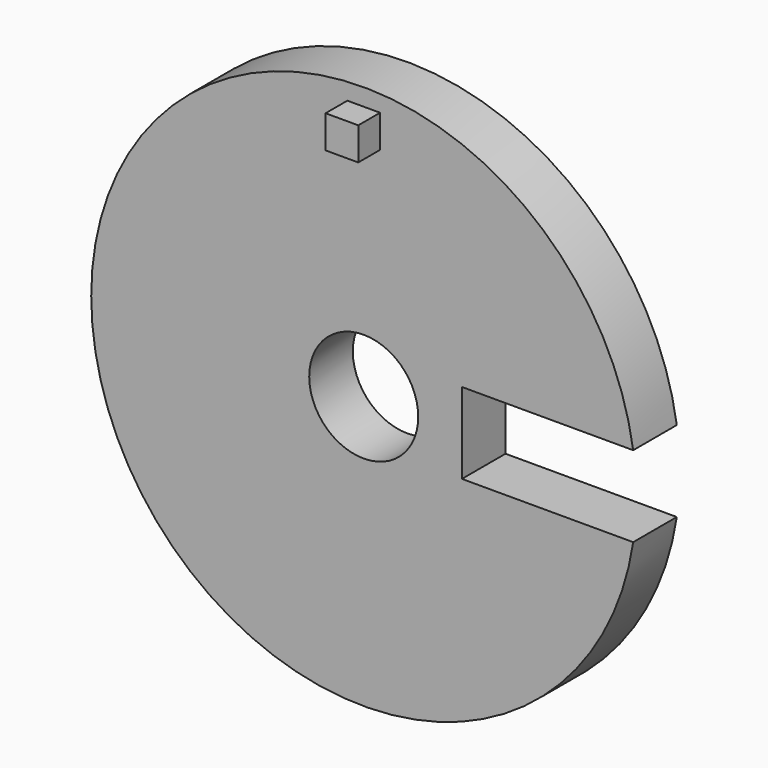
from build123d import *

# Parameters (mm, degrees)
F0_W     = 30
F0_H     = 60
F1_DEPTH = 100
F2_DEPTH = 102
F4_DEPTH = 100
F5_DEPTH = 150


# Not quite as in the source:
# - a feature of the source that left no trace in its solid (it failed there, or was rolled back) is left out
# - a feature names something its author has since deleted; it is built from what else it names


with BuildPart() as f1:
    # F0 (on Front) → F1 (new body)
    with BuildSketch(Plane.XZ):
        with BuildLine():
            Line((180.2002936602, 74.2409452796), (494.457563441, 74.2409452796))
            ThreePointArc((494.457563441, 74.2409452796), (326.2510746037, 378.8934366282), (0, 500))
            Line((0, 500), (0, 468.3614957333))
            Line((0, 468.3614957333), (30, 468.3614957333))
            Line((30, 468.3614957333), (30, 408.3614957333))
            Line((30, 408.3614957333), (0, 408.3614957333))
            Line((0, 408.3614957333), (0, 100))
            ThreePointArc((0, 100), (35.8880584042, 93.3383483033), (66.9946419051, 74.2409452796))
            Line((66.9946419051, 74.2409452796), (180.2002936602, 74.2409452796))
        make_face()
        with BuildLine():
            ThreePointArc((0, 500), (-378.8934366282, -326.2510746037), (494.457563441, -74.2409452796))
            Line((494.457563441, -74.2409452796), (180.2002936602, -74.2409452796))
            Line((180.2002936602, -74.2409452796), (66.9946419051, -74.2409452796))
            ThreePointArc((66.9946419051, -74.2409452796), (-93.3383483033, -35.8880584042), (0, 100))
            Line((0, 100), (0, 408.3614957333))
            Line((0, 408.3614957333), (-30, 408.3614957333))
            Line((-30, 408.3614957333), (-30, 468.3614957333))
            Line((-30, 468.3614957333), (0, 468.3614957333))
            Line((0, 468.3614957333), (0, 500))
        make_face()
        with BuildLine():
            Line((180.2002936602, -74.2409452796), (180.2002936602, 74.2409452796))
            Line((180.2002936602, 74.2409452796), (66.9946419051, 74.2409452796))
            ThreePointArc((66.9946419051, 74.2409452796), (91.3768684912, 40.6234895688), (100, 0))
            ThreePointArc((100, 0), (91.3768684912, -40.6234895688), (66.9946419051, -74.2409452796))
            Line((66.9946419051, -74.2409452796), (180.2002936602, -74.2409452796))
        make_face()
        with Locations((-15, 438.3614957333)):
            Rectangle(F0_W, F0_H)
    extrude(amount=F1_DEPTH)

    # F0 (on Front) → F2 (join)
    with BuildSketch(Plane.XZ):
        with Locations((15, 438.3614957333)):
            Rectangle(F0_W, F0_H)
    extrude(amount=F2_DEPTH)

    # F0 (on Front) → F4 (join)
    with BuildSketch(Plane.XZ):
        with BuildLine():
            Line((180.2002936602, 74.2409452796), (494.457563441, 74.2409452796))
            ThreePointArc((494.457563441, 74.2409452796), (326.2510746037, 378.8934366282), (0, 500))
            Line((0, 500), (0, 468.3614957333))
            Line((0, 468.3614957333), (30, 468.3614957333))
            Line((30, 468.3614957333), (30, 408.3614957333))
            Line((30, 408.3614957333), (0, 408.3614957333))
            Line((0, 408.3614957333), (0, 100))
            ThreePointArc((0, 100), (35.8880584042, 93.3383483033), (66.9946419051, 74.2409452796))
            Line((66.9946419051, 74.2409452796), (180.2002936602, 74.2409452796))
        make_face()
    extrude(amount=F4_DEPTH)

    # F0 (on Front) → F5 (join)
    with BuildSketch(Plane.XZ):
        with Locations((-15, 438.3614957333)):
            Rectangle(F0_W, F0_H)
        with Locations((15, 438.3614957333)):
            Rectangle(F0_W, F0_H)
    extrude(amount=F5_DEPTH)


solid = f1.part
